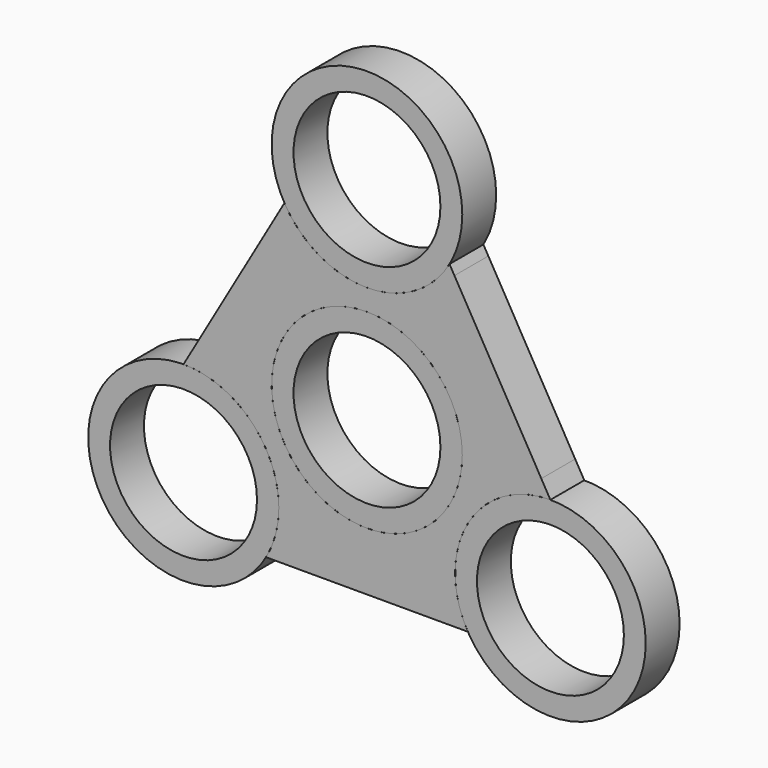
from build123d import *

# Parameters (mm, degrees)
F0_R     = 14.2875
F0_R_2   = 11.0109
F1_DEPTH = 6.35
F3_DEPTH = 6.35


with BuildPart() as f1:
    # F0 (on Front) → F1 (new body)
    with BuildSketch(Plane.XZ):
        with Locations((0, 31.75)):
            Circle(F0_R)
        with Locations((0, 31.75)):
            Circle(F0_R_2, mode=Mode.SUBTRACT)
    extrude(amount=F1_DEPTH)


with BuildPart() as f1b:
    # F0 (on Front) → F1, piece 2 (new body)
    with BuildSketch(Plane.XZ):
        Circle(F0_R)
        Circle(F0_R_2, mode=Mode.SUBTRACT)
    extrude(amount=F1_DEPTH)


with BuildPart() as f1c:
    # F0 (on Front) → F1, piece 3 (new body)
    with BuildSketch(Plane.XZ):
        with Locations((27.4963065702, -15.875)):
            Circle(F0_R)
        with Locations((27.4963065702, -15.875)):
            Circle(F0_R_2, mode=Mode.SUBTRACT)
    extrude(amount=F1_DEPTH)


with BuildPart() as f1d:
    # F0 (on Front) → F1, piece 4 (new body)
    with BuildSketch(Plane.XZ):
        with Locations((-27.4963065702, -15.875)):
            Circle(F0_R)
        with Locations((-27.4963065702, -15.875)):
            Circle(F0_R_2, mode=Mode.SUBTRACT)
    extrude(amount=F1_DEPTH)


with BuildPart() as f3:
    # F2 (on Front) → F3 (new body)
    with BuildSketch(Plane.XZ):
        with BuildLine():
            Line((-13.1735245665, 23.2202861361), (-26.7550475149, -0.3036016547))
            ThreePointArc((-26.7550475149, -0.3036016547), (-16.7530650469, 9.6043429355), (-13.1735245665, 23.2202861361))
        make_face()
        with BuildLine():
            ThreePointArc((-13.1735245665, 23.2202861361), (-16.7530650469, 9.6043429355), (-26.7550475149, -0.3036016547))
            Line((-26.7550475149, -0.3036016547), (-27.4963065702, -1.5875))
            ThreePointArc((-27.4963065702, -1.5875), (-23.7984294633, -2.0743347569), (-20.3525565702, -3.5016620434))
            Line((-20.3525565702, -3.5016620434), (-7.14375, 19.3766620434))
            ThreePointArc((-7.14375, 19.3766620434), (-10.1027881362, 21.6472118638), (-12.3733379566, 24.60625))
            Line((-12.3733379566, 24.60625), (-13.1735245665, 23.2202861361))
        make_face()
        with BuildLine():
            Line((-7.14375, 19.3766620434), (-20.3525565702, -3.5016620434))
            ThreePointArc((-20.3525565702, -3.5016620434), (-17.393518434, -5.7722118638), (-15.1229686136, -8.73125))
            Line((-15.1229686136, -8.73125), (-12.3733379566, -7.14375))
            ThreePointArc((-12.3733379566, -7.14375), (-12.3733379566, 7.14375), (0, 14.2875))
            Line((0, 14.2875), (0, 17.4625))
            ThreePointArc((0, 17.4625), (-3.6978771069, 17.9493347569), (-7.14375, 19.3766620434))
        make_face()
        with BuildLine():
            ThreePointArc((-13.2088065702, -15.875), (-13.6956413271, -19.5728771069), (-15.1229686136, -23.01875))
            Line((-15.1229686136, -23.01875), (-13.8199954558, -23.01875))
            ThreePointArc((-13.8199954558, -23.01875), (-0.0006031297, -18.5930397834), (13.8187891964, -23.01875))
            Line((13.8187891964, -23.01875), (15.1229686136, -23.01875))
            ThreePointArc((15.1229686136, -23.01875), (13.6956413271, -19.5728771069), (13.2088065702, -15.875))
            Line((13.2088065702, -15.875), (-13.2088065702, -15.875))
        make_face()
        with BuildLine():
            Line((-12.3733379566, -7.14375), (-15.1229686136, -8.73125))
            ThreePointArc((-15.1229686136, -8.73125), (-13.6956413271, -12.1771228931), (-13.2088065702, -15.875))
            Line((-13.2088065702, -15.875), (13.2088065702, -15.875))
            ThreePointArc((13.2088065702, -15.875), (13.6956413271, -12.1771228931), (15.1229686136, -8.73125))
            Line((15.1229686136, -8.73125), (12.3733379566, -7.14375))
            ThreePointArc((12.3733379566, -7.14375), (0, -14.2875), (-12.3733379566, -7.14375))
        make_face()
        with BuildLine():
            ThreePointArc((13.8187891964, -23.01875), (-0.0006031297, -18.5930397834), (-13.8199954558, -23.01875))
            Line((-13.8199954558, -23.01875), (13.8187891964, -23.01875))
        make_face()
        with BuildLine():
            ThreePointArc((7.14375, 19.3766620434), (3.6978771069, 17.9493347569), (0, 17.4625))
            Line((0, 17.4625), (0, 14.2875))
            ThreePointArc((0, 14.2875), (10.1027881362, 10.1027881362), (14.2875, 0))
            ThreePointArc((14.2875, 0), (13.8006652431, -3.6978771069), (12.3733379566, -7.14375))
            Line((12.3733379566, -7.14375), (15.1229686136, -8.73125))
            ThreePointArc((15.1229686136, -8.73125), (17.393518434, -5.7722118638), (20.3525565702, -3.5016620434))
            Line((20.3525565702, -3.5016620434), (7.14375, 19.3766620434))
        make_face()
        with BuildLine():
            ThreePointArc((12.3733379566, 24.60625), (10.1027881362, 21.6472118638), (7.14375, 19.3766620434))
            Line((7.14375, 19.3766620434), (20.3525565702, -3.5016620434))
            ThreePointArc((20.3525565702, -3.5016620434), (23.7984294633, -2.0743347569), (27.4963065702, -1.5875))
            Line((27.4963065702, -1.5875), (26.1332062792, 0.7734589597))
            ThreePointArc((26.1332062792, 0.7734589597), (16.8650497396, 10.4561422475), (13.1136783054, 23.323942901))
            Line((13.1136783054, 23.323942901), (12.3733379566, 24.60625))
        make_face()
        with BuildLine():
            Line((26.1332062792, 0.7734589597), (13.1136783054, 23.323942901))
            ThreePointArc((13.1136783054, 23.323942901), (16.8650497396, 10.4561422475), (26.1332062792, 0.7734589597))
        make_face()
    extrude(amount=F3_DEPTH)


solid = Compound([f1.part, f1b.part, f1c.part, f1d.part, f3.part])
